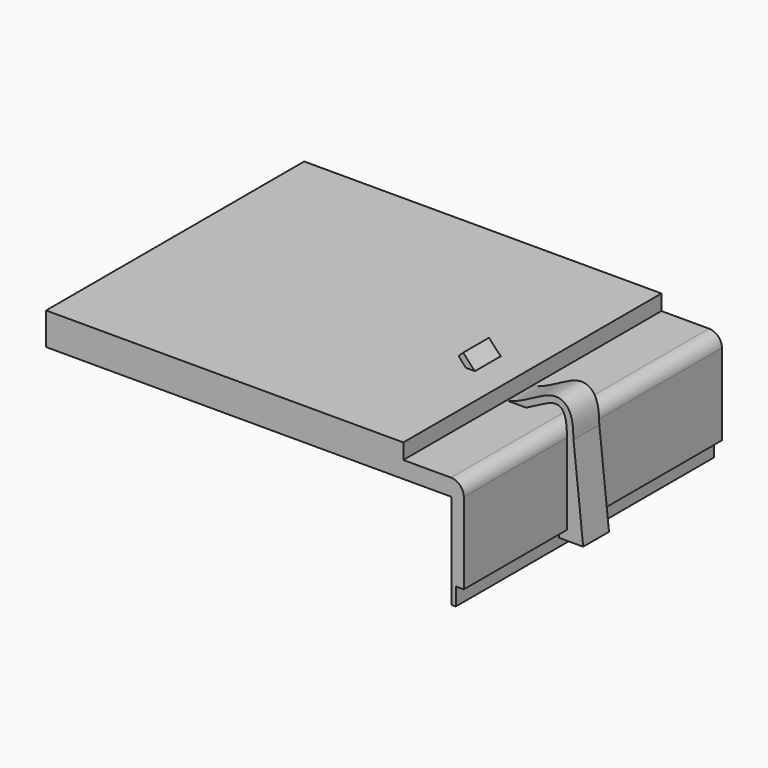
from build123d import *

# Parameters (mm, degrees)
F1_DEPTH = 50
F2_R     = 4
F4_DEPTH = 10


# Not quite as in the source:
# - the dataset's text gives a spline's control points without its knots; the knots are read off the source's solid


with BuildPart() as f1:
    # F0 (on Front) → F1 (new body, symmetric)
    with BuildSketch(Plane.XZ):
        Polygon((0, 5.5), (0, 34.7), (-18.75, 34.7), (-18.75, 39.5), (-129.4826599298, 39.5), (-129.4826599298, 29.5), (-3.8, 29.5), (-3.8, 0), (-2.5, 0), (-2.5, 5.5), align=None)
    extrude(amount=F1_DEPTH, both=True)

    # F2
    f2_edges = [f1.edges().sort_by_distance(p)[0] for p in [
        (0, 0, 34.7),
    ]]
    fillet(f2_edges, radius=F2_R)


with BuildPart() as f4:
    # F3 (on Front) → F4 (new body)
    with BuildSketch(Plane.XZ):
        with BuildLine():
            Line((0, 30.7), (0, 5.5))
            Line((0, 5.5), (-1.5, 5.5))
            Line((-1.5, 5.5), (-1.5, 7))
            Line((-1.5, 7), (-2.5, 7))
            Line((-2.5, 7), (-2.5, 5.5))
            Line((-2.5, 5.5), (-2.5, 2.5))
            Line((-2.5, 2.5), (5, 2.5))
            Line((5, 2.5), (2, 30.7))
            add(Edge.make_bspline(
                [(2, 30.7), (2, 31.7663755094), (1.9197978856, 33.6815229202), (1.560050438, 36.0024950572), (1.0325239491, 37.5777989644), (0.4158888599, 38.6629640394), (-0.1636126536, 39.3793411079), (-0.8646567386, 39.9695560734), (-1.6592021315, 40.3955071637), (-2.4904020482, 40.6421178896), (-3.5805366392, 40.7585096187), (-4.8446996517, 40.6044084525), (-6.228916873, 40.1740055139), (-7.3247518132, 39.7044300401), (-8.1785645119, 39.2998972581), (-9.0326113969, 38.8755002829), (-10.096764527, 38.3183652887), (-11.7962518236, 37.4052131626), (-13.9106977139, 36.2897970194), (-16.3926786988, 35.2017320437), (-18.3509918097, 34.6630955174), (-19.8166550492, 34.5167284053), (-20.6917970101, 34.5499347509), (-21.3766716144, 34.6571924904), (-21.8821148851, 34.7794442799), (-22.4057251629, 34.9520837377), (-23.1251886297, 35.2478795474), (-24.0538174781, 35.7349619931), (-25.1834777576, 36.4780606848), (-26.3004948953, 37.3423008268), (-27.7421408169, 38.6023216567), (-29.0715230137, 39.9406021799), (-30.2243827664, 41.1936677419), (-30.9885209637, 42.052275421), (-31.6443353319, 42.7955467899), (-32.0096009958, 43.1975262649), (-32.1846689975, 43.3795967395)],
                knots=[0, 0, 0, 0, 0.03125, 0.0625, 0.09375, 0.109375, 0.125, 0.140625, 0.15625, 0.171875, 0.1875, 0.21875, 0.25, 0.28125, 0.296875, 0.3125, 0.34375, 0.375, 0.4375, 0.5, 0.5625, 0.59375, 0.625, 0.640625, 0.65625, 0.671875, 0.6875, 0.71875, 0.75, 0.78125, 0.8125, 0.875, 0.90625, 0.9375, 0.96875, 1, 1, 1, 1], degree=3))
            Line((-32.1846689975, 43.3795967395), (-33.6263341869, 41.993378329))
            add(Edge.make_bspline(
                [(0, 30.7), (0, 39.9784169766), (-7.3101929171, 38.6941557742), (-22.175657359, 27.5773311116), (-32.0087713963, 40.311115311), (-33.6263341869, 41.993378329)],
                knots=[0, 0, 0, 0, 0.2853917714, 0.6513245985, 1, 1, 1, 1], degree=3))
        make_face()
    extrude(amount=F4_DEPTH)


solid = Compound([f1.part, f4.part])
